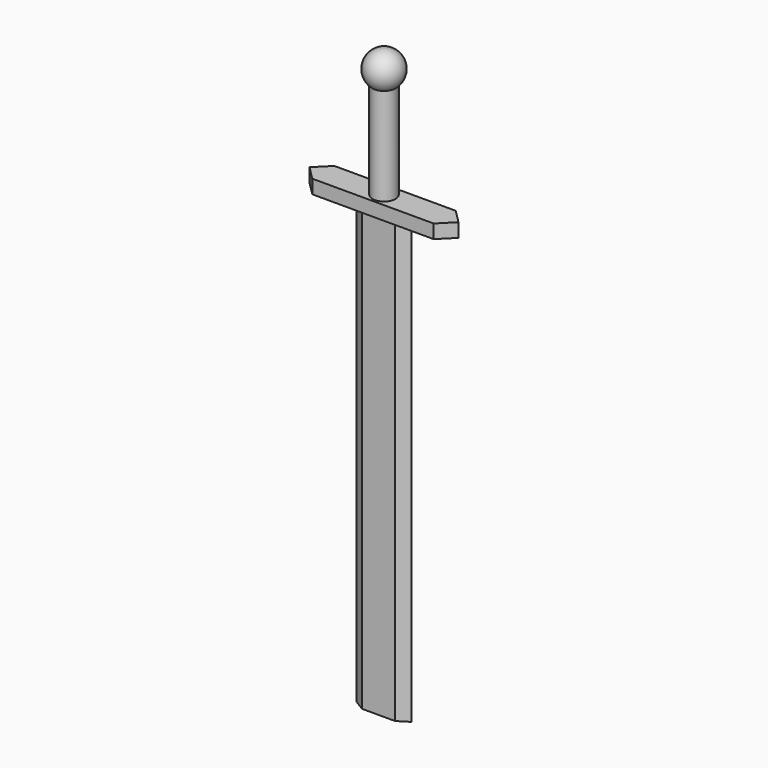
from build123d import *

# Parameters (mm, degrees)
F1_DEPTH    = 76.2
F2_W        = 38.1
F2_H        = 6.35
F3_DEPTH    = 3.175
F4_T1_DEPTH = 29.3032991577
F5_R        = 2.6614768155
F6_DEPTH    = 25.4
F10_DEPTH   = 25.4


# Not quite as in the source:
# - a fillet or chamfer that OpenCascade refuses, or shapes differently, is made with other operations: its cross-section is extruded or revolved along the edge and cut away or added


with BuildPart() as f1:
    # F0 (on Top) → F1 (new body)
    with BuildSketch(Plane.XY):
        Polygon((0, 1.5875), (-3.81, 1.5875), (-6.35, 0), (-3.81, -1.5875), (0, -1.5875), (3.81, -1.5875), (6.35, 0), (3.81, 1.5875), align=None)
    extrude(amount=F1_DEPTH)

    # F2 (on face) → F3 (join)
    with BuildSketch(Plane.XY.offset(76.2)):
        Rectangle(F2_W, F2_H)
    extrude(amount=F3_DEPTH)

    # F4: chamfer of 5.08 on 4 edges, made by hand

    # F4_s2 → F4_t1 (cut)
    with BuildSketch(Plane.XY.offset(63.1358504211)):
        Polygon((19.05, 1.905), (13.97, -3.175), (19.05, -3.175), align=None)
        Polygon((13.97, 3.175), (19.05, -1.905), (19.05, 3.175), align=None)
        Polygon((-19.05, 1.905), (-13.97, -3.175), (-19.05, -3.175), align=None)
        Polygon((-13.97, 3.175), (-19.05, -1.905), (-19.05, 3.175), align=None)
    extrude(amount=F4_T1_DEPTH, mode=Mode.SUBTRACT)

    # F5 (on face) → F6 (join)
    with BuildSketch(Plane.XY.offset(79.375)):
        Circle(F5_R)
    extrude(amount=F6_DEPTH)

    # F7 (on Front) → F9 (revolve)
    with BuildSketch(Plane.XZ):
        with BuildLine():
            Line((0, 108.979212298), (0, 100.7914969782))
            ThreePointArc((0, 100.7914969782), (4.0938576599, 104.8853546381), (0, 108.979212298))
        make_face()
    revolve(axis=Axis((0, 0, 105.8157756925), (0, 0, 1)))

    # F10 (add): a face of the model
    f10_faces = [f1.faces().sort_by_distance(p)[0] for p in [
        (0, 0, 0),
    ]]
    extrude(f10_faces, amount=F10_DEPTH)


solid = f1.part
